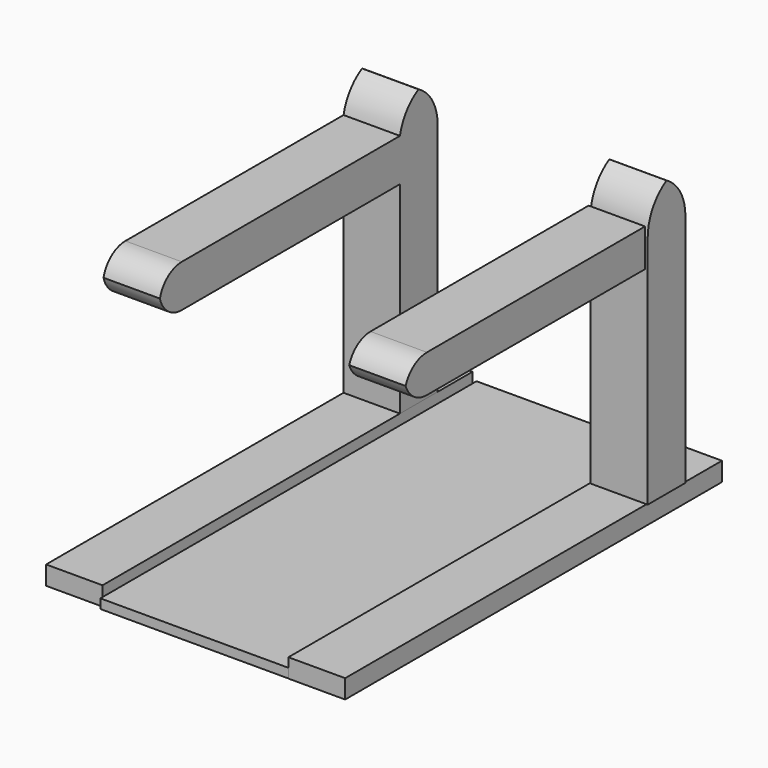
from build123d import *

# Parameters (mm, degrees)
F0_W          = 100
F0_H          = 250
F1_DEPTH      = 5
F2_W          = 30
F2_H          = 245.8441516644
F3_DEPTH      = 10
F2_W_2        = 30.1613137126
F2_H_2        = 250.4182979465
F4_W          = 30
F4_H          = 25.0615030527
F5_DEPTH      = 150
F4_W_2        = 30.434358865
F4_H_2        = 25.0502228737
F6_W          = 30
F6_H          = 22.6044723392
F7_DEPTH      = 160
F6_H_2        = 20
F8_T1_DEPTH   = 152.4744871392
F8_T3_DEPTH   = 155
F8_2_T1_DEPTH = 155.434358865
F9_T1_DEPTH   = 105
F9_2_T1_DEPTH = 105


# Not quite as in the source:
# - a fillet or chamfer that OpenCascade refuses, or shapes differently, is made with other operations: its cross-section is extruded or revolved along the edge and cut away or added


with BuildPart() as f1:
    # F0 (on Top) → F1 (new body)
    with BuildSketch(Plane.XY):
        with Locations((8.8387416875, 61.2532682717)):
            Rectangle(F0_W, F0_H)
    extrude(amount=F1_DEPTH)


with BuildPart() as f3:
    # F2 (on Top) → F3 (new body)
    with BuildSketch(Plane.XY):
        with Locations((-56.7995943129, 61.3852031529)):
            Rectangle(F2_W, F2_H)
    extrude(amount=F3_DEPTH)


with BuildPart() as f3b:
    # F2 (on Top) → F3, piece 2 (new body)
    with BuildSketch(Plane.XY):
        with Locations((73.9655904472, 61.3852031529)):
            Rectangle(F2_W_2, F2_H_2)
    extrude(amount=F3_DEPTH)


with BuildPart() as f5:
    # F4 (on face) → F5 (new body)
    with BuildSketch(Plane.XY.offset(10)):
        with Locations((-56.7995943129, 148.6918106675)):
            Rectangle(F4_W, F4_H)
    extrude(amount=F5_DEPTH)

    # F6 (on face) → F7 (join)
    with BuildSketch(Plane.XZ.offset(-136.1610591412)):
        with Locations((-56.7995943129, 128.6977638304)):
            Rectangle(F6_W, F6_H)
    extrude(amount=F7_DEPTH)

    # F8: fillet of radius 25 on 2 edges, made by hand

    # F8_s2 → F8_t1 (cut)
    with BuildSketch(Plane.YZ.offset(-133.0368378825)):
        with BuildLine():
            ThreePointArc((160.655956569, 160), (144.8445682681, 154.364916731), (136.1610591412, 140))
            Line((136.1610591412, 140), (136.1610591412, 160))
            Line((136.1610591412, 160), (160.655956569, 160))
        make_face()
    extrude(amount=F8_T1_DEPTH, mode=Mode.SUBTRACT)

    # F8_s4 → F8_t3 (cut)
    with BuildSketch(Plane.YZ.offset(-134.2995943129)):
        with BuildLine():
            ThreePointArc((161.2225621939, 135), (153.9002317235, 152.6776695297), (136.2225621939, 160))
            Line((136.2225621939, 160), (161.2225621939, 160))
            Line((161.2225621939, 160), (161.2225621939, 135))
        make_face()
    extrude(amount=F8_T3_DEPTH, mode=Mode.SUBTRACT)

    # F9: fillet of radius 15 on 2 edges, made by hand

    # F9_s2 → F9_t1 (cut)
    with BuildSketch(Plane.YZ.offset(-109.2995943129)):
        with BuildLine():
            ThreePointArc((-23.8389408588, 125), (-19.4455425766, 135.6066017178), (-8.8389408588, 140))
            Line((-8.8389408588, 140), (-23.8389408588, 140))
            Line((-23.8389408588, 140), (-23.8389408588, 125))
        make_face()
        with BuildLine():
            ThreePointArc((-8.8389408588, 117.3955276608), (-19.4455425766, 121.788925943), (-23.8389408588, 132.3955276608))
            Line((-23.8389408588, 132.3955276608), (-23.8389408588, 117.3955276608))
            Line((-23.8389408588, 117.3955276608), (-8.8389408588, 117.3955276608))
        make_face()
    extrude(amount=F9_T1_DEPTH, mode=Mode.SUBTRACT)


with BuildPart() as f5b:
    # F4 (on face) → F5, piece 2 (new body)
    with BuildSketch(Plane.XY.offset(10)):
        with Locations((74.460586533, 149.00611341)):
            Rectangle(F4_W_2, F4_H_2)
    extrude(amount=F5_DEPTH)

    # F8#2: fillet of radius 25 on 2 edges, made by hand

    # F8_2_s2 → F8_2_t1 (cut)
    with BuildSketch(Plane.YZ.offset(-3.2565928996)):
        with BuildLine():
            ThreePointArc((136.4810019732, 135), (143.8033324435, 152.6776695297), (161.4810019732, 160))
            Line((161.4810019732, 160), (136.4810019732, 160))
            Line((136.4810019732, 160), (136.4810019732, 135))
        make_face()
        with BuildLine():
            ThreePointArc((161.5312248468, 135), (154.2088943765, 152.6776695297), (136.5312248468, 160))
            Line((136.5312248468, 160), (161.5312248468, 160))
            Line((161.5312248468, 160), (161.5312248468, 135))
        make_face()
    extrude(amount=F8_2_T1_DEPTH, mode=Mode.SUBTRACT)


with BuildPart() as f7:
    # F6 (on face) → F7, piece 2 (new body)
    with BuildSketch(Plane.XZ.offset(-136.1610591412)):
        with Locations((73.5199929774, 130)):
            Rectangle(F6_W, F6_H_2)
    extrude(amount=F7_DEPTH)

    # F9#2: fillet of radius 15 on 2 edges, made by hand

    # F9_2_s2 → F9_2_t1 (cut)
    with BuildSketch(Plane.YZ.offset(21.0199929774)):
        with BuildLine():
            ThreePointArc((-8.8389408588, 140), (-19.4455425766, 135.6066017178), (-23.8389408588, 125))
            Line((-23.8389408588, 125), (-23.8389408588, 140))
            Line((-23.8389408588, 140), (-8.8389408588, 140))
        make_face()
        with BuildLine():
            ThreePointArc((-8.8389408588, 120), (-19.4455425766, 124.3933982822), (-23.8389408588, 135))
            Line((-23.8389408588, 135), (-23.8389408588, 120))
            Line((-23.8389408588, 120), (-8.8389408588, 120))
        make_face()
    extrude(amount=F9_2_T1_DEPTH, mode=Mode.SUBTRACT)


solid = Compound([f1.part, f3.part, f3b.part, f5.part, f5b.part, f7.part])
